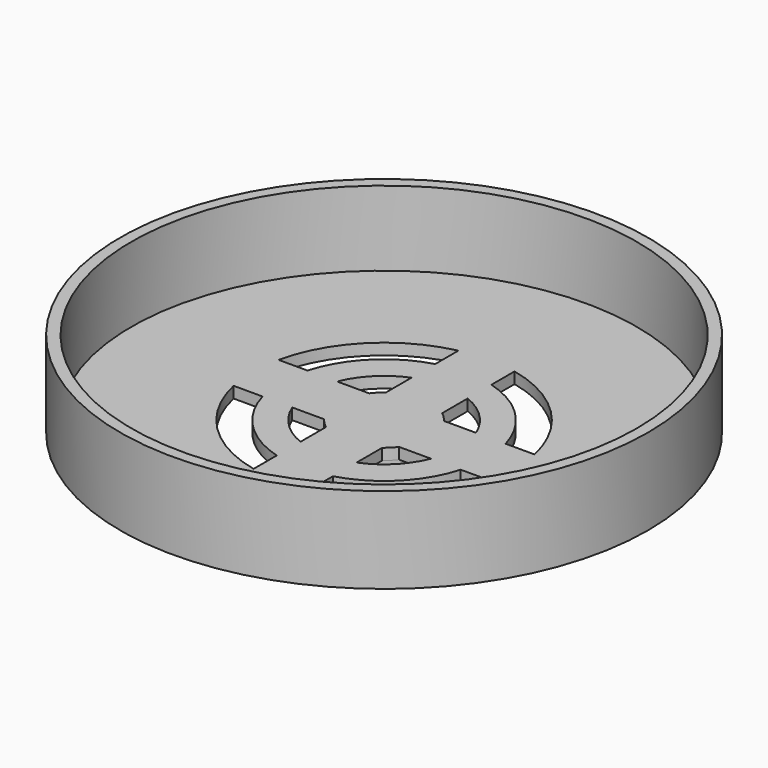
from build123d import *

# Parameters (mm, degrees)
F0_R     = 28.2
F1_DEPTH = 9.2
F2_T     = -1.2
F4_DEPTH = 9.201
F5_R     = 5
F6_DEPTH = 4


# Not quite as in the source:
# - after a boolean that leaves OpenCascade's solid faulty, fix() repairs it


with BuildPart() as f1:
    # F0 (on Top) → F1 (new body)
    with BuildSketch(Plane.XY):
        Circle(F0_R)
    extrude(amount=F1_DEPTH)

    # F2
    f2_openings = [f1.faces().sort_by_distance(p)[0] for p in [
        (0, 0, 9.2),
    ]]
    offset(amount=F2_T, openings=f2_openings)

    # F3 (on face) → F4 (cut, through all)
    with BuildSketch(Plane(origin=(0, 0, 0), x_dir=(1, 0, 0), z_dir=(0, 0, -1))):
        with BuildLine():
            ThreePointArc((4, -3), (3.5355339059, -3.5355339059), (3, -4))
            Line((3, -4), (3, -7.4161984871))
            ThreePointArc((3, -7.4161984871), (5.6568542495, -5.6568542495), (7.4161984871, -3))
            Line((7.4161984871, -3), (4, -3))
        make_face()
        with BuildLine():
            ThreePointArc((10.5830052443, -3), (7.7781745931, -7.7781745931), (3, -10.5830052443))
            Line((3, -10.5830052443), (3, -13.6747943312))
            ThreePointArc((3, -13.6747943312), (9.8994949366, -9.8994949366), (13.6747943312, -3))
            Line((13.6747943312, -3), (10.5830052443, -3))
        make_face()
        with BuildLine():
            ThreePointArc((-13.6747943312, -3), (-9.8994949366, -9.8994949366), (-3, -13.6747943312))
            Line((-3, -13.6747943312), (-3, -10.5830052443))
            ThreePointArc((-3, -10.5830052443), (-7.7781745931, -7.7781745931), (-10.5830052443, -3))
            Line((-10.5830052443, -3), (-13.6747943312, -3))
        make_face()
        with BuildLine():
            ThreePointArc((-4, 3), (-3.5355339059, 3.5355339059), (-3, 4))
            Line((-3, 4), (-3, 7.4161984871))
            ThreePointArc((-3, 7.4161984871), (-5.6568542495, 5.6568542495), (-7.4161984871, 3))
            Line((-7.4161984871, 3), (-4, 3))
        make_face()
        with BuildLine():
            ThreePointArc((-10.5830052443, 3), (-7.7781745931, 7.7781745931), (-3, 10.5830052443))
            Line((-3, 10.5830052443), (-3, 13.6747943312))
            ThreePointArc((-3, 13.6747943312), (-9.8994949366, 9.8994949366), (-13.6747943312, 3))
            Line((-13.6747943312, 3), (-10.5830052443, 3))
        make_face()
        with BuildLine():
            Line((10.5830052443, 3), (13.6747943312, 3))
            ThreePointArc((13.6747943312, 3), (9.8994949366, 9.8994949366), (3, 13.6747943312))
            Line((3, 13.6747943312), (3, 10.5830052443))
            ThreePointArc((3, 10.5830052443), (7.7781745931, 7.7781745931), (10.5830052443, 3))
        make_face()
        with BuildLine():
            Line((4, 3), (7.4161984871, 3))
            ThreePointArc((7.4161984871, 3), (5.6568542495, 5.6568542495), (3, 7.4161984871))
            Line((3, 7.4161984871), (3, 4))
            ThreePointArc((3, 4), (3.5355339059, 3.5355339059), (4, 3))
        make_face()
        with BuildLine():
            Line((-4, -3), (-7.4161984871, -3))
            ThreePointArc((-7.4161984871, -3), (-5.6568542495, -5.6568542495), (-3, -7.4161984871))
            Line((-3, -7.4161984871), (-3, -4))
            ThreePointArc((-3, -4), (-3.5355339059, -3.5355339059), (-4, -3))
        make_face()
    extrude(amount=-F4_DEPTH, mode=Mode.SUBTRACT)

    # F5 (on face) → F6 (join)
    with BuildSketch(Plane(origin=(0, 0, 0), x_dir=(1, 0, 0), z_dir=(0, 0, -1))):
        Circle(F5_R)
    extrude(amount=F6_DEPTH)

    add(f1.part.fix(), mode=Mode.REPLACE)


solid = f1.part
